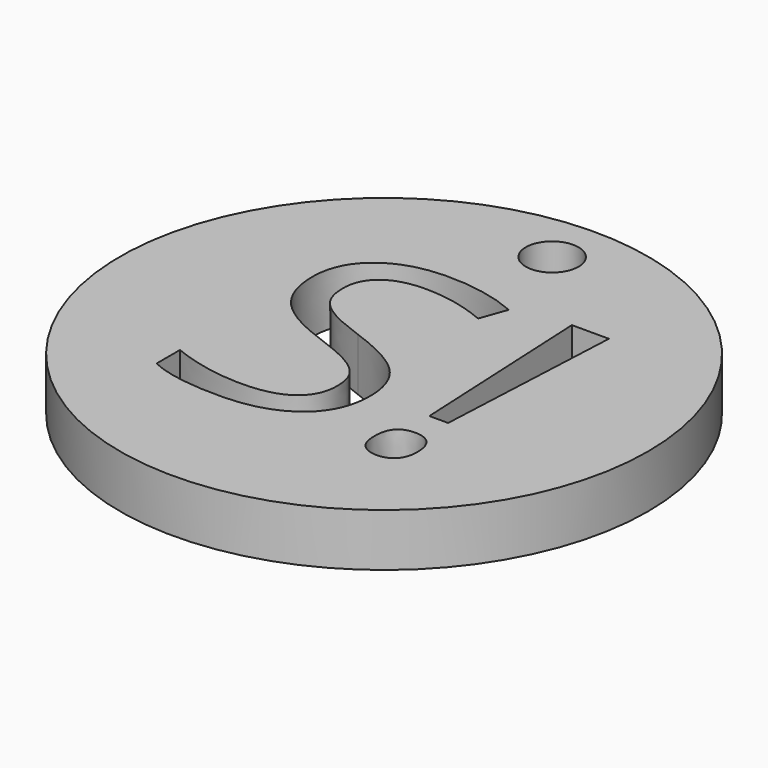
from build123d import *

# Parameters (mm, degrees)
F0_R         = 15
F1_DEPTH     = 3
F2_R         = 1.5
F2_TEXT_SIZE = 20.8333333333
F3_DEPTH     = 3.001


# Not quite as in the source:
# - Text() gives the source's letters only with a copy of the font that has no kerning and outlines rounded to 1/6400 em; it was checked with that copy


with BuildPart() as f1:
    # F0 (on Top) → F1 (new body)
    with BuildSketch(Plane.XY):
        Circle(F0_R)
    extrude(amount=F1_DEPTH)

    # F2 (on face) → F3 (cut, through all)
    with BuildSketch(Plane.XY.offset(3)):
        with Locations((0, 11.9408629835)):
            Circle(F2_R)
        with Locations((-8.3919270833, -7.5)):
            Text('S!', F2_TEXT_SIZE, font='Open Sans', text_align=(TextAlign.LEFT, TextAlign.BOTTOM))
    extrude(amount=-F3_DEPTH, mode=Mode.SUBTRACT)


solid = f1.part
